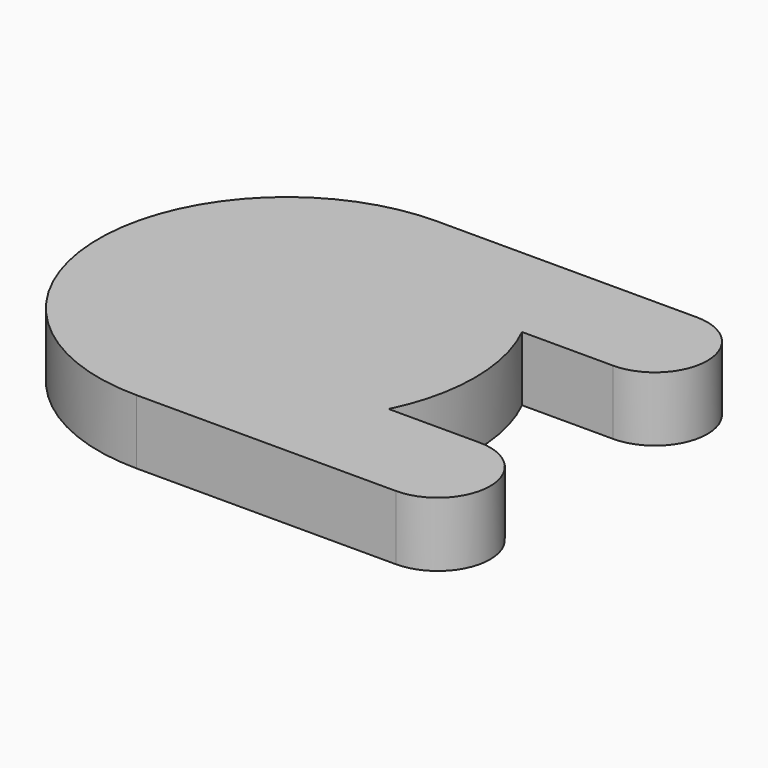
from build123d import *

# Parameters (mm, degrees)
F1_DEPTH = 25.4


with BuildPart() as f1:
    # F0 (on Top) → F1 (new body)
    with BuildSketch(Plane.XY):
        with BuildLine():
            ThreePointArc((0.0883997278, 32.8236170641), (-13.058763384, 37.4885196208), (-20.2230135431, 49.4585962042))
            ThreePointArc((-20.2230135431, 49.4585962042), (-53.4333511512, 0), (-20.2230135431, -49.4585962042))
            ThreePointArc((-20.2230135431, -49.4585962042), (-13.0929285798, -37.5165620637), (0, -32.8234274819))
            Line((0, -32.8234274819), (42.1633208321, -32.8234274819))
            ThreePointArc((42.1633208321, -32.8234274819), (50.5373651023, -17.3521682727), (53.4333511512, 0))
            ThreePointArc((53.4333511512, 0), (50.5373260912, 17.3522818904), (42.1631732449, 32.8236170641))
            Line((42.1631732449, 32.8236170641), (0.0883997278, 32.8236170641))
        make_face()
        with BuildLine():
            ThreePointArc((0, -32.8234274819), (-13.0929285798, -37.5165620637), (-20.2230135431, -49.4585962042))
            ThreePointArc((-20.2230135431, -49.4585962042), (-10.3049618346, -52.4302467745), (0, -53.4333511512))
            ThreePointArc((0, -53.4333511512), (10.3049618346, -52.4302467745), (20.2230135431, -49.4585962042))
            ThreePointArc((20.2230135431, -49.4585962042), (13.0929285798, -37.5165620637), (0, -32.8234274819))
        make_face()
        with BuildLine():
            ThreePointArc((0, -32.8234274819), (13.0929285798, -37.5165620637), (20.2230135431, -49.4585962042))
            ThreePointArc((20.2230135431, -49.4585962042), (32.2830588513, -42.5784819651), (42.1633208321, -32.8234274819))
            Line((42.1633208321, -32.8234274819), (0, -32.8234274819))
        make_face()
        with BuildLine():
            Line((0, -53.4333511512), (20.6099236693, -53.4333511512))
            ThreePointArc((20.6099236693, -53.4333511512), (20.5129680829, -51.436580237), (20.2230135431, -49.4585962042))
            ThreePointArc((20.2230135431, -49.4585962042), (10.3049618346, -52.4302467745), (0, -53.4333511512))
        make_face()
        with BuildLine():
            Line((20.6099236693, -53.4333511512), (51.2570339651, -53.4333511512))
            ThreePointArc((51.2570339651, -53.4333511512), (59.7096740135, -43.7854013954), (66.3703936593, -32.8234274819))
            Line((66.3703936593, -32.8234274819), (42.1633208321, -32.8234274819))
            ThreePointArc((42.1633208321, -32.8234274819), (32.2830588513, -42.5784819651), (20.2230135431, -49.4585962042))
            ThreePointArc((20.2230135431, -49.4585962042), (20.5129680829, -51.436580237), (20.6099236693, -53.4333511512))
        make_face()
        with BuildLine():
            ThreePointArc((102.2053944331, -32.8234274819), (87.6319776468, -38.8599343649), (81.5954707638, -53.4333511512))
            Line((81.5954707638, -53.4333511512), (102.2053944331, -53.4333511512))
            Line((102.2053944331, -53.4333511512), (102.2053944331, -32.8234274819))
        make_face()
        with BuildLine():
            ThreePointArc((20.6099236693, 53.4333511512), (14.5734167863, 68.0067679375), (0, 74.0432748205))
            ThreePointArc((0, 74.0432748205), (-15.9167890876, 66.526279731), (-20.2230135431, 49.4585962042))
            ThreePointArc((-20.2230135431, 49.4585962042), (-10.3049618346, 52.4302467745), (0, 53.4333511512))
            Line((0, 53.4333511512), (20.6099236693, 53.4333511512))
        make_face()
        with BuildLine():
            ThreePointArc((51.2570339651, 53.4333511512), (27.6226921414, 68.6978414873), (0, 74.0432748205))
            ThreePointArc((0, 74.0432748205), (14.5734167863, 68.0067679375), (20.6099236693, 53.4333511512))
            Line((20.6099236693, 53.4333511512), (51.2570339651, 53.4333511512))
        make_face()
        with BuildLine():
            ThreePointArc((81.5954707638, -53.4333511512), (87.6319776468, -68.0067679375), (102.2053944331, -74.0432748205))
            Line((102.2053944331, -74.0432748205), (102.2053944331, -53.4333511512))
            Line((102.2053944331, -53.4333511512), (81.5954707638, -53.4333511512))
        make_face()
        with BuildLine():
            Line((102.2053944331, 74.0432748205), (0, 74.0432748205))
            ThreePointArc((0, 74.0432748205), (27.6226921414, 68.6978414873), (51.2570339651, 53.4333511512))
            Line((51.2570339651, 53.4333511512), (81.5954707638, 53.4333511512))
            ThreePointArc((81.5954707638, 53.4333511512), (87.6319776468, 68.0067679375), (102.2053944331, 74.0432748205))
        make_face()
        with BuildLine():
            ThreePointArc((-20.2230135431, -49.4585962042), (-15.9167890876, -66.526279731), (0, -74.0432748205))
            ThreePointArc((0, -74.0432748205), (14.5734167863, -68.0067679375), (20.6099236693, -53.4333511512))
            Line((20.6099236693, -53.4333511512), (0, -53.4333511512))
            ThreePointArc((0, -53.4333511512), (-10.3049618346, -52.4302467745), (-20.2230135431, -49.4585962042))
        make_face()
        with BuildLine():
            ThreePointArc((122.8153181024, 53.4333511512), (116.7788112194, 68.0067679375), (102.2053944331, 74.0432748205))
            Line((102.2053944331, 74.0432748205), (102.2053944331, 53.4333511512))
            Line((102.2053944331, 53.4333511512), (102.2053944331, 32.8236170641))
            Line((102.2053944331, 32.8236170641), (102.2053944331, 32.8234274819))
            ThreePointArc((102.2053944331, 32.8234274819), (116.7788112194, 38.8599343649), (122.8153181024, 53.4333511512))
        make_face()
        with BuildLine():
            Line((102.2053944331, 53.4333511512), (102.2053944331, 74.0432748205))
            ThreePointArc((102.2053944331, 74.0432748205), (87.6319776468, 68.0067679375), (81.5954707638, 53.4333511512))
            Line((81.5954707638, 53.4333511512), (102.2053944331, 53.4333511512))
        make_face()
        with BuildLine():
            ThreePointArc((20.6099236693, -53.4333511512), (14.5734167863, -68.0067679375), (0, -74.0432748205))
            ThreePointArc((0, -74.0432748205), (27.6226921414, -68.6978414873), (51.2570339651, -53.4333511512))
            Line((51.2570339651, -53.4333511512), (20.6099236693, -53.4333511512))
        make_face()
        with BuildLine():
            ThreePointArc((51.2570339651, -53.4333511512), (27.6226921414, -68.6978414873), (0, -74.0432748205))
            Line((0, -74.0432748205), (102.2053944331, -74.0432748205))
            ThreePointArc((102.2053944331, -74.0432748205), (87.6319776468, -68.0067679375), (81.5954707638, -53.4333511512))
            Line((81.5954707638, -53.4333511512), (51.2570339651, -53.4333511512))
        make_face()
        with BuildLine():
            ThreePointArc((-20.2230135431, 49.4585962042), (-15.9167890876, 66.526279731), (0, 74.0432748205))
            ThreePointArc((0, 74.0432748205), (-74.0432748205, 0), (0, -74.0432748205))
            ThreePointArc((0, -74.0432748205), (-15.9167890876, -66.526279731), (-20.2230135431, -49.4585962042))
            ThreePointArc((-20.2230135431, -49.4585962042), (-53.4333511512, 0), (-20.2230135431, 49.4585962042))
        make_face()
        with BuildLine():
            ThreePointArc((66.3703936593, -32.8234274819), (59.7096740135, -43.7854013954), (51.2570339651, -53.4333511512))
            Line((51.2570339651, -53.4333511512), (81.5954707638, -53.4333511512))
            ThreePointArc((81.5954707638, -53.4333511512), (87.6319776468, -38.8599343649), (102.2053944331, -32.8234274819))
            Line((102.2053944331, -32.8234274819), (66.3703936593, -32.8234274819))
        make_face()
        with BuildLine():
            Line((102.2053944331, 32.8236170641), (102.1169947054, 32.8236170641))
            ThreePointArc((102.1169947054, 32.8236170641), (102.1611944676, 32.8234748775), (102.2053944331, 32.8234274819))
            Line((102.2053944331, 32.8234274819), (102.2053944331, 32.8236170641))
        make_face()
        with BuildLine():
            Line((102.2053944331, -53.4333511512), (102.2053944331, -74.0432748205))
            ThreePointArc((102.2053944331, -74.0432748205), (116.7788112194, -68.0067679375), (122.8153181024, -53.4333511512))
            ThreePointArc((122.8153181024, -53.4333511512), (116.7788112194, -38.8599343649), (102.2053944331, -32.8234274819))
            Line((102.2053944331, -32.8234274819), (102.2053944331, -53.4333511512))
        make_face()
        with BuildLine():
            Line((102.2053944331, 53.4333511512), (81.5954707638, 53.4333511512))
            ThreePointArc((81.5954707638, 53.4333511512), (87.6007570653, 38.891221974), (102.1169947054, 32.8236170641))
            Line((102.1169947054, 32.8236170641), (102.2053944331, 32.8236170641))
            Line((102.2053944331, 32.8236170641), (102.2053944331, 53.4333511512))
        make_face()
        with BuildLine():
            Line((81.5954707638, 53.4333511512), (51.2570339651, 53.4333511512))
            ThreePointArc((51.2570339651, 53.4333511512), (59.7096114785, 43.7854866736), (66.3702999012, 32.8236170641))
            Line((66.3702999012, 32.8236170641), (102.1169947054, 32.8236170641))
            ThreePointArc((102.1169947054, 32.8236170641), (87.6007570653, 38.891221974), (81.5954707638, 53.4333511512))
        make_face()
        with BuildLine():
            ThreePointArc((66.3702999012, 32.8236170641), (59.7096114785, 43.7854866736), (51.2570339651, 53.4333511512))
            Line((51.2570339651, 53.4333511512), (20.6099236693, 53.4333511512))
            ThreePointArc((20.6099236693, 53.4333511512), (20.5129680829, 51.436580237), (20.2230135431, 49.4585962042))
            ThreePointArc((20.2230135431, 49.4585962042), (32.2829631266, 42.5785545435), (42.1631732449, 32.8236170641))
            Line((42.1631732449, 32.8236170641), (66.3702999012, 32.8236170641))
        make_face()
        with BuildLine():
            ThreePointArc((20.2230135431, 49.4585962042), (20.5129680829, 51.436580237), (20.6099236693, 53.4333511512))
            Line((20.6099236693, 53.4333511512), (0, 53.4333511512))
            ThreePointArc((0, 53.4333511512), (10.3049618346, 52.4302467745), (20.2230135431, 49.4585962042))
        make_face()
        with BuildLine():
            ThreePointArc((0, 53.4333511512), (-10.3049618346, 52.4302467745), (-20.2230135431, 49.4585962042))
            ThreePointArc((-20.2230135431, 49.4585962042), (-13.058763384, 37.4885196208), (0.0883997278, 32.8236170641))
            ThreePointArc((0.0883997278, 32.8236170641), (13.1270335572, 37.5446777126), (20.2230135431, 49.4585962042))
            ThreePointArc((20.2230135431, 49.4585962042), (10.3049618346, 52.4302467745), (0, 53.4333511512))
        make_face()
        with BuildLine():
            ThreePointArc((74.0432748205, 0), (72.0995176879, 16.8542604501), (66.3702999012, 32.8236170641))
            Line((66.3702999012, 32.8236170641), (42.1631732449, 32.8236170641))
            ThreePointArc((42.1631732449, 32.8236170641), (50.5373260912, 17.3522818904), (53.4333511512, 0))
            Line((53.4333511512, 0), (74.0432748205, 0))
        make_face()
        with BuildLine():
            Line((42.1633208321, -32.8234274819), (66.3703936593, -32.8234274819))
            ThreePointArc((66.3703936593, -32.8234274819), (72.0995417593, -16.8541574765), (74.0432748205, 0))
            Line((74.0432748205, 0), (53.4333511512, 0))
            ThreePointArc((53.4333511512, 0), (50.5373651023, -17.3521682727), (42.1633208321, -32.8234274819))
        make_face()
        with BuildLine():
            ThreePointArc((42.1631732449, 32.8236170641), (32.2829631266, 42.5785545435), (20.2230135431, 49.4585962042))
            ThreePointArc((20.2230135431, 49.4585962042), (13.1270335572, 37.5446777126), (0.0883997278, 32.8236170641))
            Line((0.0883997278, 32.8236170641), (42.1631732449, 32.8236170641))
        make_face()
    extrude(amount=F1_DEPTH)


solid = f1.part
